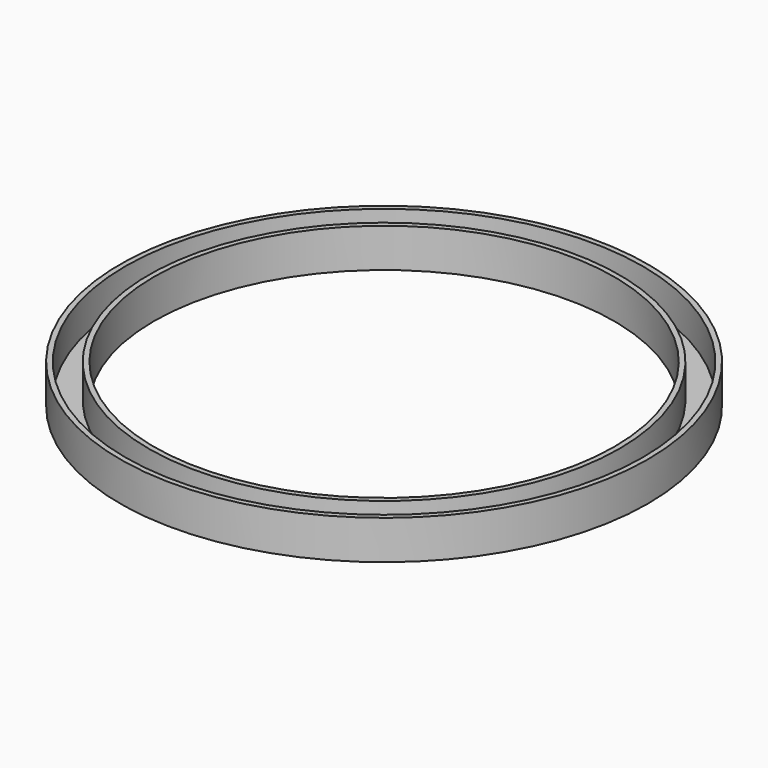
from build123d import *

# Parameters (mm, degrees)
F0_R     = 101.5
F1_DEPTH = 15
F2_R     = 88.5
F3_DEPTH = 15.001
F4_T     = -2


# Not quite as in the source:
# - a feature names something its author has since deleted; it is built from what else it names


with BuildPart() as f1:
    # F0 (on Top) → F1 (new body)
    with BuildSketch(Plane.XY):
        Circle(F0_R)
    extrude(amount=F1_DEPTH)

    # F2 (on face) → F3 (cut, through all)
    with BuildSketch(Plane.XY.offset(15)):
        Circle(F2_R)
    extrude(amount=-F3_DEPTH, mode=Mode.SUBTRACT)

    # F4
    f4_openings = [f1.faces().sort_by_distance(p)[0] for p in [
        (-98.629146, 0, 15),
    ]]
    offset(amount=F4_T, openings=f4_openings)


solid = f1.part
